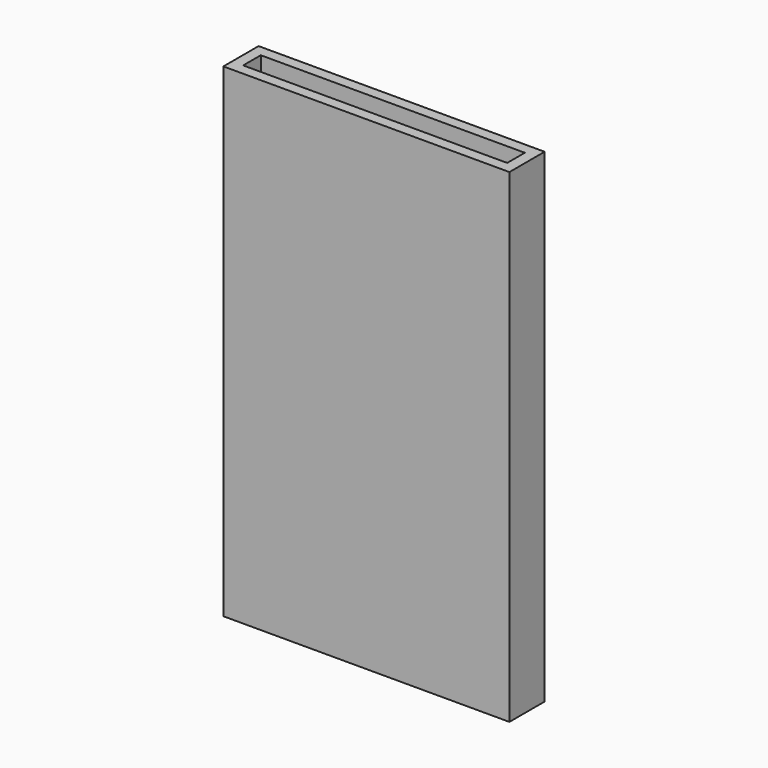
from build123d import *

# Parameters (mm, degrees)
F0_W         = 52
F0_H         = 8
F0_W_2       = 48
F0_H_2       = 4
F1_DEPTH     = 88
F2_W         = 48
F2_H         = 4
F3_DEPTH     = 2
F4_TEXT_SIZE = 4.4538639167
F5_DEPTH     = 1


# Not quite as in the source:
# - Text() gives the source's letters only with a copy of the font that has no kerning and outlines rounded to 1/6400 em; it was checked with that copy


with BuildPart() as f1:
    # F0 (on Top) → F1 (new body)
    with BuildSketch(Plane.XY):
        with Locations((2.9437100291, -0.0558064356)):
            Rectangle(F0_W, F0_H)
        with Locations((2.9437100291, -0.0558064356)):
            Rectangle(F0_W_2, F0_H_2, mode=Mode.SUBTRACT)
    extrude(amount=F1_DEPTH)

    # F2 (on face) → F3 (join)
    with BuildSketch(Plane(origin=(0, 0, 0), x_dir=(1, 0, 0), z_dir=(0, 0, -1))):
        with Locations((2.9437100291, 0.0558064356)):
            Rectangle(F2_W, F2_H)
    extrude(amount=-F3_DEPTH)

    # F4 (on face) → F5 (cut)
    with BuildSketch(Plane(origin=(0, 3.9441935644, 0), x_dir=(-1, 0, 0), z_dir=(0, 1, 0))):
        with Locations(Location((2.9871217128, 59.0672824471), (0, 0, -90))):
            Text('Rita Bragadesto', F4_TEXT_SIZE, font='Open Sans', text_align=(TextAlign.LEFT, TextAlign.BOTTOM))
        with Locations(Location((-3.070133214, 61.3818998513), (0, 0, -90))):
            Text('Training Specialist', F4_TEXT_SIZE, font='Open Sans', text_align=(TextAlign.LEFT, TextAlign.BOTTOM))
        with Locations(Location((-9.1273881407, 81.0561477873), (0, 0, -90))):
            Text('Pharmaceutical Products Development', F4_TEXT_SIZE, font='Open Sans', text_align=(TextAlign.LEFT, TextAlign.BOTTOM))
    extrude(amount=-F5_DEPTH, mode=Mode.SUBTRACT)


solid = f1.part
